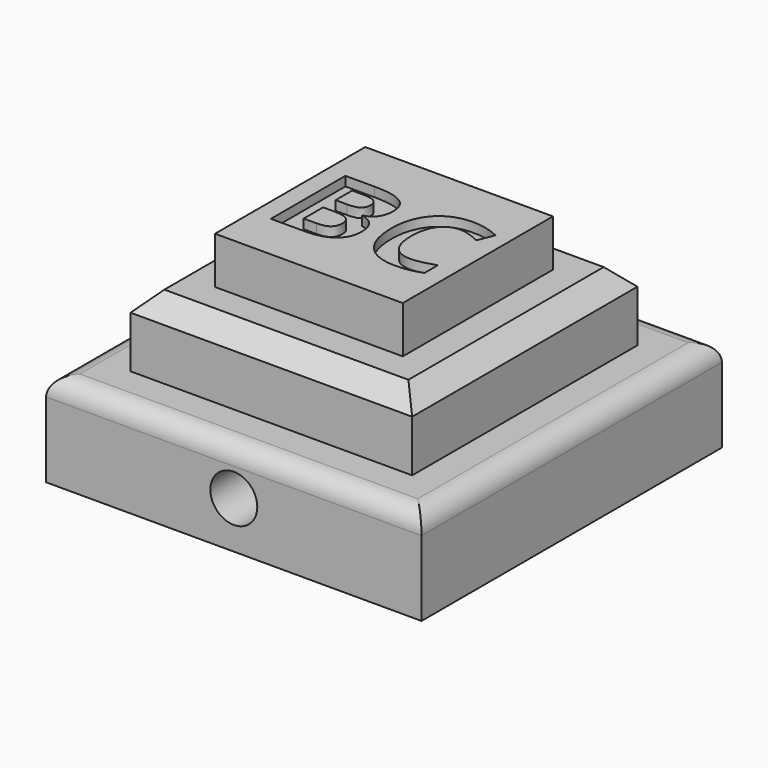
from build123d import *

# Parameters (mm, degrees)
F0_W          = 101.6
F0_H          = 101.6
F1_DEPTH      = 25.4
F2_W          = 76.2
F2_H          = 76.2
F3_DEPTH      = 19.05
F4_W          = 50.8
F4_H          = 50.8
F5_DEPTH      = 12.7
F6_R          = 6.35
F7_DEPTH      = 181.864
F8_R          = 5.08
F9_SIZE       = 5.08
F10_TEXT_SIZE = 35.2777777778
F11_DEPTH     = 2.54


# Not quite as in the source:
# - Text() gives the source's letters only with a copy of the font that has no kerning and outlines rounded to 1/6400 em; it was checked with that copy


with BuildPart() as f1:
    # F0 (on Top) → F1 (new body)
    with BuildSketch(Plane.XY):
        with Locations((50.8, 50.8)):
            Rectangle(F0_W, F0_H)
    extrude(amount=F1_DEPTH)

    # F2 (on face) → F3 (join)
    with BuildSketch(Plane.XY.offset(25.4)):
        with Locations((50.8, 50.8)):
            Rectangle(F2_W, F2_H)
    extrude(amount=F3_DEPTH)

    # F4 (on face) → F5 (join)
    with BuildSketch(Plane.XY.offset(44.45)):
        with Locations((50.8, 50.8)):
            Rectangle(F4_W, F4_H)
    extrude(amount=F5_DEPTH)

    # F6 (on face) → F7 (cut)
    with BuildSketch(Plane.XZ):
        with Locations((50.8, 12.7)):
            Circle(F6_R)
    extrude(amount=-F7_DEPTH, mode=Mode.SUBTRACT)

    # F8
    f8_edges = [f1.edges().sort_by_distance(p)[0] for p in [
        (101.6, 50.8, 25.4),
        (50.8, 0, 25.4),
        (0, 50.8, 25.4),
        (50.8, 101.6, 25.4),
    ]]
    fillet(f8_edges, radius=F8_R)

    # F9
    f9_edges = [f1.edges().sort_by_distance(p)[0] for p in [
        (88.9, 50.8, 44.45),
        (50.8, 12.7, 44.45),
        (50.8, 88.9, 44.45),
        (12.7, 50.8, 44.45),
    ]]
    chamfer(f9_edges, length=F9_SIZE)

    # F10 (on face) → F11 (cut)
    with BuildSketch(Plane.XY.offset(57.15)):
        with Locations((27.1859375, 38.1)):
            Text('BC', F10_TEXT_SIZE, font='Open Sans', font_style=FontStyle.BOLD, text_align=(TextAlign.LEFT, TextAlign.BOTTOM))
    extrude(amount=-F11_DEPTH, mode=Mode.SUBTRACT)


solid = f1.part
